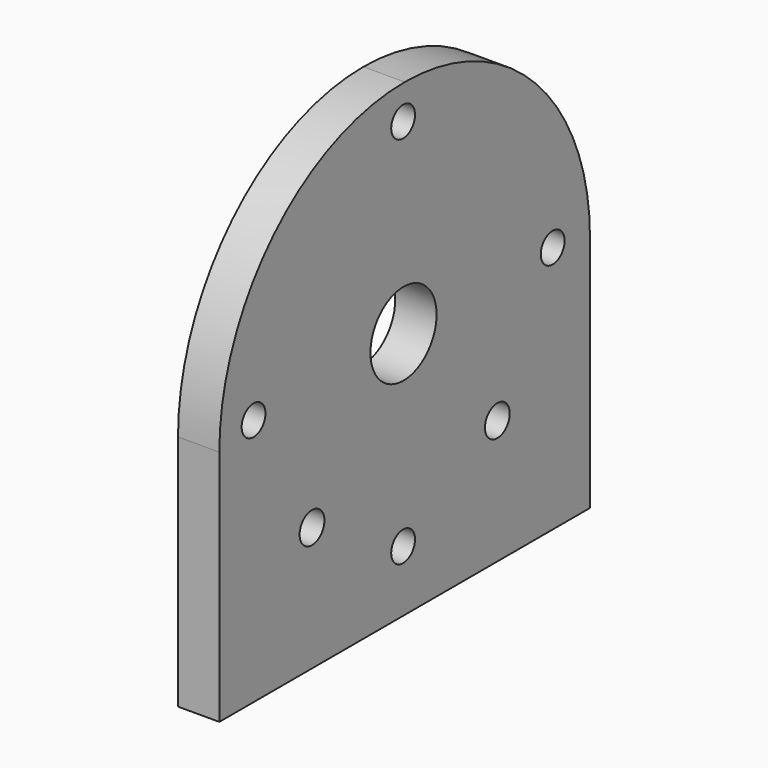
from build123d import *

# Parameters (mm, degrees)
F0_R     = 2.286
F0_R_2   = 6.35
F1_DEPTH = 6.35


# Not quite as in the source:
# - ends of sketch curves that miss each other by under 0.0002 mm in the source are joined


with BuildPart() as f1:
    # F0 (on Right) → F1 (new body)
    with BuildSketch(Plane.YZ):
        with BuildLine():
            Line((-35.36227718, -1.6545656172), (-35.36227718, -38.1239391863))
            Line((-35.36227718, -38.1239391863), (-17.5702907145, -38.1239391863))
            Line((-17.5702907145, -38.1239391863), (0.221695751, -38.1239391863))
            Line((0.221695751, -38.1239391863), (18.0136822164, -38.1239391863))
            Line((18.0136822164, -38.1239391863), (35.8056686819, -38.1239391863))
            Line((35.8056686819, -38.1239391863), (35.8056686819, -1.6545656172))
            ThreePointArc((35.8056686819, -1.6545656172), (25.3839554031, 23.5071029235), (0.22312282, 33.9308342683))
            Line((0.22312282, 33.9308342683), (0.2202686819, 33.9308343828))
            ThreePointArc((0.2202686819, 33.9308343828), (-24.9405639012, 23.5071029235), (-35.36227718, -1.6545656172))
        make_face()
        with Locations((-0.074788043, -28.7147061436)):
            Circle(F0_R, mode=Mode.SUBTRACT)
        with BuildLine():
            ThreePointArc((-15.1890407145, -19.0739391863), (-15.8864926918, -20.757737209), (-17.5702907145, -21.4551891863))
            ThreePointArc((-17.5702907145, -21.4551891863), (-19.2540887372, -17.3901411636), (-15.1890407145, -19.0739391863))
        make_face(mode=Mode.SUBTRACT)
        with BuildLine():
            ThreePointArc((20.3949322164, -19.0739391863), (19.6974802391, -20.757737209), (18.0136822164, -21.4551891863))
            ThreePointArc((18.0136822164, -21.4551891863), (16.3298841937, -17.3901411636), (20.3949322164, -19.0739391863))
        make_face(mode=Mode.SUBTRACT)
        with Locations((-28.7894941866, 0)):
            Circle(F0_R, mode=Mode.SUBTRACT)
        Circle(F0_R_2, mode=Mode.SUBTRACT)
        with Locations((-0.0747941866, 28.7147)):
            Circle(F0_R, mode=Mode.SUBTRACT)
        with Locations((28.639911957, -6.1436e-06)):
            Circle(F0_R, mode=Mode.SUBTRACT)
    extrude(amount=F1_DEPTH)


solid = f1.part
